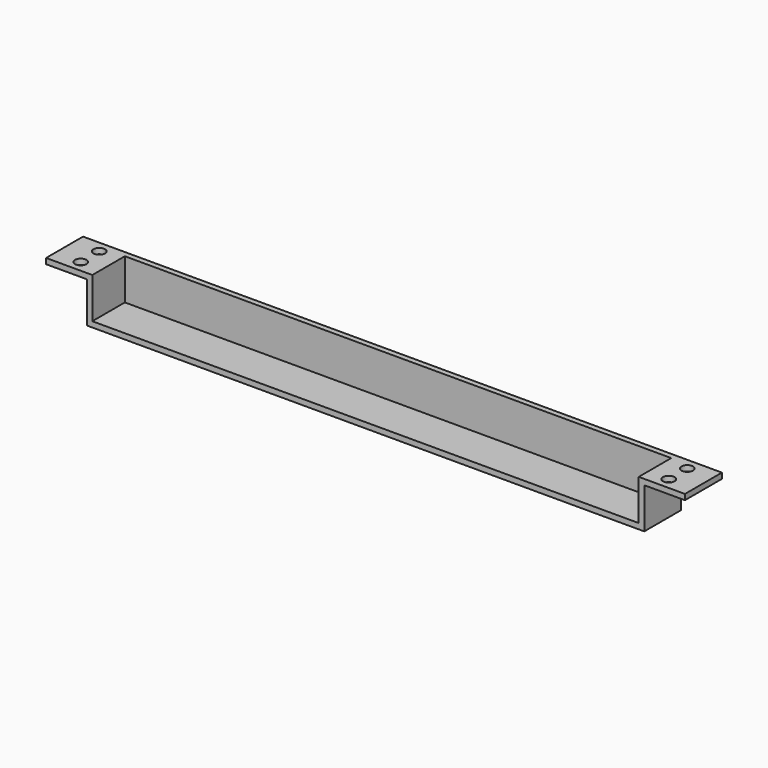
from build123d import *

# Parameters (mm, degrees)
F1_DEPTH = 295.5
F3_DEPTH = 50
F5_D     = 12.5


# Not quite as in the source:
# - a pattern or mirror of a feature is missing from the dataset's text; its kind, count and spacing are read off the source's solid


with BuildPart() as f1:
    # F0 (on Right) → F1 (new body, symmetric)
    with BuildSketch(Plane.YZ):
        Polygon((0, 6), (0, 0), (50, 0), (50, 50), (44, 50), (44, 6), align=None)
    extrude(amount=F1_DEPTH, both=True)

    # F2 (on face) → F3 (join)
    with BuildSketch(Plane(origin=(0, 50, 0), x_dir=(-1, 0, 0), z_dir=(0, 1, 0))):
        Polygon((-301.5, 0), (-295.5, 0), (-295.5, 50), (-345.5, 50), (-345.5, 44), (-301.5, 44), align=None)
    f3 = extrude(amount=-F3_DEPTH)

    # F3_copies: F3 across plane
    add(f3.mirror(Plane(origin=(0, 0, 0), x_dir=(0, 0, -1), z_dir=(-1, 0, 0))))

    # F5 (through all)
    with Locations(Plane.XY.offset(50)):
        with Locations((318, 37.5), (318, 12.5)):
            f5 = Hole(F5_D / 2)

    # F5_copies: F5 across plane
    add(f5.mirror(Plane(origin=(0, 0, 0), x_dir=(0, 0, -1), z_dir=(-1, 0, 0))), mode=Mode.SUBTRACT)


solid = f1.part
